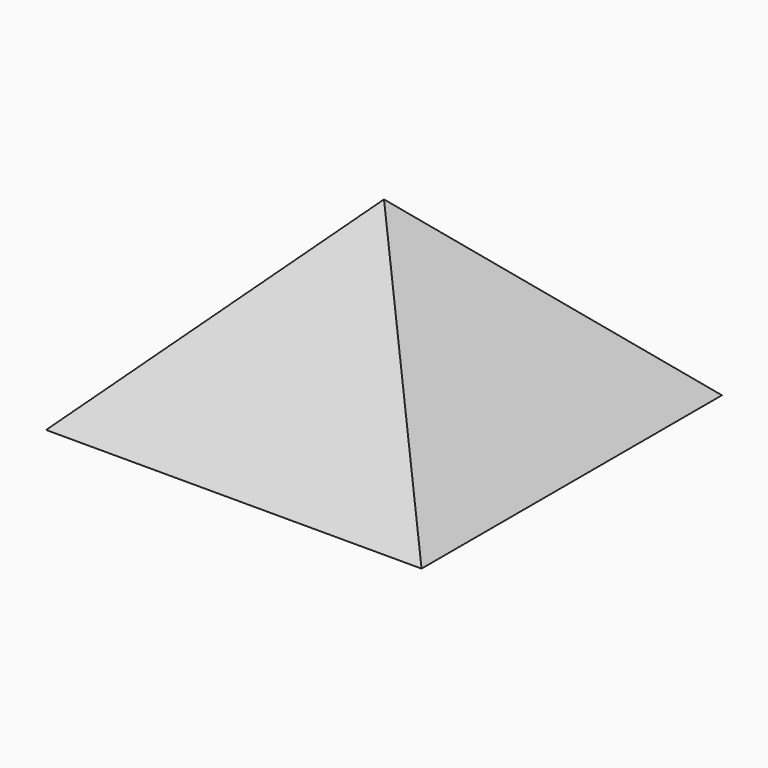
from build123d import *

# Parameters (mm, degrees)
F0_W     = 7000
F0_H     = 7000
F1_DEPTH = 7000
F2_SIZE  = 3499.99999
F3_DEPTH = 3500


# Not quite as in the source:
# - a fillet or chamfer is up to 0.001 mm smaller than in the source, because OpenCascade refuses the exact size


with BuildPart() as f1:
    # F0 (on Top) → F1 (new body)
    with BuildSketch(Plane.XY):
        with Locations((3500, 3500)):
            Rectangle(F0_W, F0_H)
    extrude(amount=F1_DEPTH)

    # F2 (size 3500 in the source; OpenCascade refuses exactly that, so slightly less here)
    f2_edges = [f1.edges().sort_by_distance(p)[0] for p in [
        (3500, 0, 7000),
        (7000, 3500, 7000),
        (3500, 7000, 7000),
        (0, 3500, 7000),
    ]]
    chamfer(f2_edges, length=F2_SIZE)

    # F3 (cut): a face of the model
    f3_faces = [f1.faces().sort_by_distance(p)[0] for p in [
        (3500, 3500, 0),
    ]]
    extrude(f3_faces, amount=-F3_DEPTH, mode=Mode.SUBTRACT)


solid = f1.part
